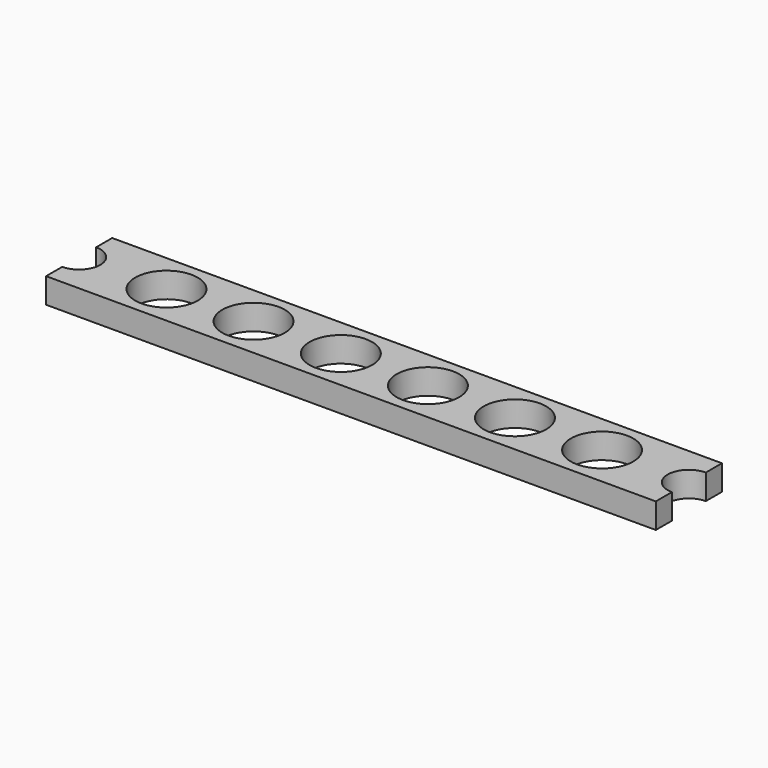
from build123d import *

# Parameters (mm, degrees)
F0_R     = 31
F1_DEPTH = 25


# Not quite as in the source:
# - ends of sketch curves that miss each other by under 0.0002 mm in the source are joined


with BuildPart() as f1:
    # F0 (on Top) → F1 (new body)
    with BuildSketch(Plane.XY):
        with BuildLine():
            Line((-302.7446055809, 143.0378559404), (-302.7446061336, 123.0378559404))
            Line((-302.7446061336, 123.0378559404), (302.2563133603, 123.0378559404))
            Line((302.2563133603, 123.0378559404), (302.2563133603, 143.0378559404))
            ThreePointArc((302.2563133603, 143.0378559404), (281.2558506145, 164.0373893883), (302.2553878584, 185.0378521342))
            Line((302.2553878584, 185.0378521342), (302.2553878585, 205.0378483381))
            Line((302.2553878585, 205.0378483381), (-302.7446121415, 205.0378559404))
            Line((-302.7446121415, 205.0378559404), (-302.7446123928, 185.0378559404))
            ThreePointArc((-302.7446123928, 185.0378559404), (-281.7446089869, 164.0378593463), (-302.7446055809, 143.0378559404))
        make_face()
        with Locations((-216.3446089869, 164.3591374159)):
            Circle(F0_R, mode=Mode.SUBTRACT)
        with Locations((-129.9446089869, 164.3591374159)):
            Circle(F0_R, mode=Mode.SUBTRACT)
        with Locations((-43.3446089869, 164.3591374159)):
            Circle(F0_R, mode=Mode.SUBTRACT)
        with Locations((43.0553910131, 164.3591374159)):
            Circle(F0_R, mode=Mode.SUBTRACT)
        with Locations((129.4553910131, 164.3591374159)):
            Circle(F0_R, mode=Mode.SUBTRACT)
        with Locations((215.8553910131, 164.3591374159)):
            Circle(F0_R, mode=Mode.SUBTRACT)
    extrude(amount=F1_DEPTH)


solid = f1.part
